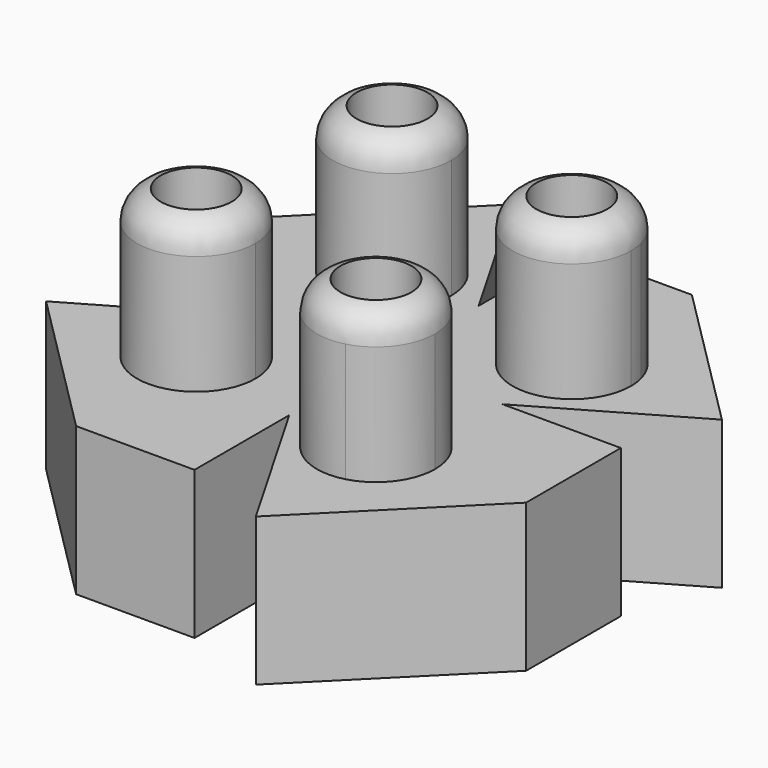
from build123d import *

# Parameters (mm, degrees)
F1_DEPTH = 25
F2_DEPTH = 50
F3_R     = 6
F4_DEPTH = 50
F5_DEPTH = 50


# Not quite as in the source:
# - a fillet or chamfer that OpenCascade refuses, or shapes differently, is made with other operations: its cross-section is extruded or revolved along the edge and cut away or added


with BuildPart() as f1:
    # F0 (on Top) → F1 (new body)
    with BuildSketch(Plane.XY):
        Polygon((0, -20), (0, 0), (-20, 0), (-45.3589838486, -14.6410161514), (-20, -40), (0, -40), align=None)
        with BuildLine():
            ThreePointArc((-10, -14.6410161514), (-18.6986197214, -24.5559750202), (-29.6612818741, -17.2216425383))
            ThreePointArc((-29.6612818741, -17.2216425383), (-21.3013802786, -4.7260572825), (-10, -14.6410161514))
        make_face(mode=Mode.SUBTRACT)
        Polygon((-20, 0), (0, 0), (0, 20), (-14.6410161514, 45.3589838486), (-40, 20), (-40, 0), align=None)
        with BuildLine():
            ThreePointArc((-4.6410161514, 20), (-20.7317359828, 12.0688505288), (-17.2216425383, 29.6612818741))
            ThreePointArc((-17.2216425383, 29.6612818741), (-8.5502963199, 27.9311494712), (-4.6410161514, 20))
        make_face(mode=Mode.SUBTRACT)
        Polygon((0, 20), (0, 0), (20, 0), (45.3589838486, 14.6410161514), (20, 40), (0, 40), align=None)
        with BuildLine():
            ThreePointArc((30, 14.6410161514), (10.0850411312, 13.3396358728), (29.6612818741, 17.2216425383))
            ThreePointArc((29.6612818741, 17.2216425383), (29.9149588688, 15.9423964299), (30, 14.6410161514))
        make_face(mode=Mode.SUBTRACT)
        Polygon((20, 0), (0, 0), (0, -20), (14.6410161514, -45.3589838486), (40, -20), (40, 0), align=None)
        with BuildLine():
            ThreePointArc((24.6410161514, -20), (22.5721656226, -26.0907198315), (17.2216425383, -29.6612818741))
            ThreePointArc((17.2216425383, -29.6612818741), (6.7098666802, -13.9092801685), (24.6410161514, -20))
        make_face(mode=Mode.SUBTRACT)
        with BuildLine():
            ThreePointArc((-10, -14.6410161514), (-21.3013802786, -4.7260572825), (-29.6612818741, -17.2216425383))
            ThreePointArc((-29.6612818741, -17.2216425383), (-18.6986197214, -24.5559750202), (-10, -14.6410161514))
        make_face()
        with BuildLine():
            ThreePointArc((-4.6410161514, 20), (-8.5502963199, 27.9311494712), (-17.2216425383, 29.6612818741))
            ThreePointArc((-17.2216425383, 29.6612818741), (-20.7317359828, 12.0688505288), (-4.6410161514, 20))
        make_face()
        with BuildLine():
            ThreePointArc((30, 14.6410161514), (29.9149588688, 15.9423964299), (29.6612818741, 17.2216425383))
            ThreePointArc((29.6612818741, 17.2216425383), (10.0850411312, 13.3396358728), (30, 14.6410161514))
        make_face()
        with BuildLine():
            ThreePointArc((24.6410161514, -20), (6.7098666802, -13.9092801685), (17.2216425383, -29.6612818741))
            ThreePointArc((17.2216425383, -29.6612818741), (22.5721656226, -26.0907198315), (24.6410161514, -20))
        make_face()
    extrude(amount=F1_DEPTH)

    # F0 (on Top) → F2 (join)
    with BuildSketch(Plane.XY):
        with BuildLine():
            ThreePointArc((24.6410161514, -20), (6.7098666802, -13.9092801685), (17.2216425383, -29.6612818741))
            ThreePointArc((17.2216425383, -29.6612818741), (22.5721656226, -26.0907198315), (24.6410161514, -20))
        make_face()
        with BuildLine():
            ThreePointArc((-10, -14.6410161514), (-21.3013802786, -4.7260572825), (-29.6612818741, -17.2216425383))
            ThreePointArc((-29.6612818741, -17.2216425383), (-18.6986197214, -24.5559750202), (-10, -14.6410161514))
        make_face()
        with BuildLine():
            ThreePointArc((-4.6410161514, 20), (-8.5502963199, 27.9311494712), (-17.2216425383, 29.6612818741))
            ThreePointArc((-17.2216425383, 29.6612818741), (-20.7317359828, 12.0688505288), (-4.6410161514, 20))
        make_face()
        with BuildLine():
            ThreePointArc((30, 14.6410161514), (29.9149588688, 15.9423964299), (29.6612818741, 17.2216425383))
            ThreePointArc((29.6612818741, 17.2216425383), (10.0850411312, 13.3396358728), (30, 14.6410161514))
        make_face()
    extrude(amount=F2_DEPTH)

    # F3 (on face) → F4 (cut)
    with BuildSketch(Plane.XY.offset(50)):
        with Locations((-14.6410161514, 20)):
            Circle(F3_R)
    extrude(amount=-F4_DEPTH, mode=Mode.SUBTRACT)

    # F3 (on face) → F5 (cut)
    with BuildSketch(Plane.XY.offset(50)):
        with Locations((20, 14.6410161514)):
            Circle(F3_R)
        with Locations((14.6410161514, -20)):
            Circle(F3_R)
        with Locations((-20, -14.6410161514)):
            Circle(F3_R)
        with Locations((-14.6410161514, 20)):
            Circle(F3_R)
    extrude(amount=-F5_DEPTH, mode=Mode.SUBTRACT)

    # F6: fillet of radius 5 on 4 edges, made by hand

    # F6_s1 → F6_t2 (revolve, cut)
    with BuildSketch(Plane.XZ.offset(14.6410161514)):
        with BuildLine():
            ThreePointArc((-10, 45.1010205144), (-11.1270166538, 48.2632981746), (-14, 50))
            Line((-14, 50), (-10, 50))
            Line((-10, 50), (-10, 45.1010205144))
        make_face()
    revolve(axis=Axis((-20, -14.6410161514, 50), (0, 0, 1)), mode=Mode.SUBTRACT)

    # F6_s3 → F6_t4 (revolve, cut)
    with BuildSketch(Plane.XZ.offset(-20)):
        with BuildLine():
            ThreePointArc((-4.6410161514, 45.1010205144), (-5.7680328052, 48.2632981746), (-8.6410161514, 50))
            Line((-8.6410161514, 50), (-4.6410161514, 50))
            Line((-4.6410161514, 50), (-4.6410161514, 45.1010205144))
        make_face()
    revolve(axis=Axis((-14.6410161514, 20, 50), (0, 0, 1)), mode=Mode.SUBTRACT)

    # F6_s5 → F6_t6 (revolve, cut)
    with BuildSketch(Plane(origin=(8.6795464871, 2.3183949069, 0), x_dir=(0, 0, 1), z_dir=(-0.9661281874, -0.2580626387, 0))):
        with BuildLine():
            ThreePointArc((45.1010205144, -33.1008630094), (48.2632981746, -31.9738463556), (50, -29.1008630094))
            Line((50, -29.1008630094), (50, -33.1008630094))
            Line((50, -33.1008630094), (45.1010205144, -33.1008630094))
        make_face()
    revolve(axis=Axis((14.6410161514, -20, 50), (0, 0, 1)), mode=Mode.SUBTRACT)

    # F6_s7 → F6_t8 (revolve, cut)
    with BuildSketch(Plane.XZ.offset(-14.6410161514)):
        with BuildLine():
            ThreePointArc((30, 45.1010205144), (28.8729833462, 48.2632981746), (26, 50))
            Line((26, 50), (30, 50))
            Line((30, 50), (30, 45.1010205144))
        make_face()
    revolve(axis=Axis((20, 14.6410161514, 50), (0, 0, 1)), mode=Mode.SUBTRACT)


solid = f1.part
